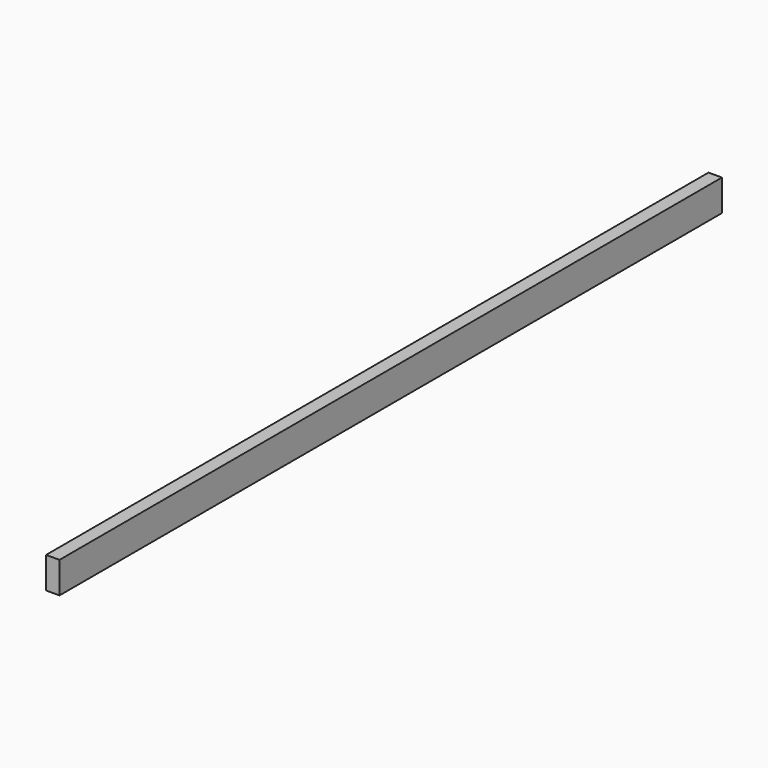
from build123d import *

# Parameters (mm, degrees)
F1_W     = 38.1
F1_H     = 88.9
F2_DEPTH = 2349.5


# Not quite as in the source:
# - a variable given as a bare number and used for a length is read in inches; the dataset says mm whatever the document's units were


with BuildPart() as f2:
    # F1 (on Front) → F2 (new body)
    with BuildSketch(Plane.XZ):
        with Locations((19.05, 44.45)):
            Rectangle(F1_W, F1_H)
    extrude(amount=F2_DEPTH)


solid = f2.part
